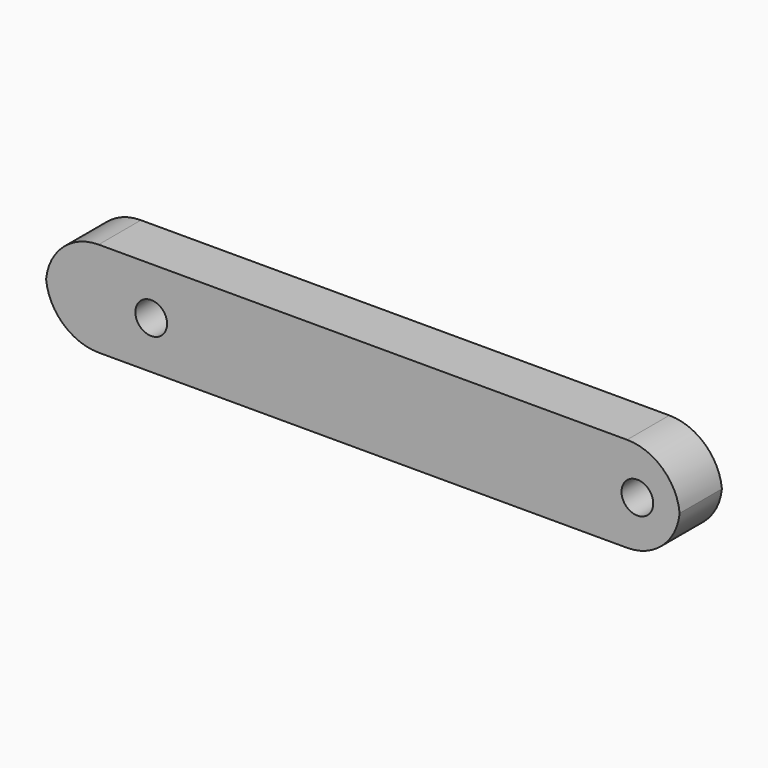
from build123d import *

# Parameters (mm, degrees)
F0_W        = 60
F0_H        = 9
F1_DEPTH    = 5
F2_T1_DEPTH = 30
F3_R        = 1.5
F4_DEPTH    = 12.5


# Not quite as in the source:
# - a fillet or chamfer that OpenCascade refuses, or shapes differently, is made with other operations: its cross-section is extruded or revolved along the edge and cut away or added


with BuildPart() as f1:
    # F0 (on Front) → F1 (new body)
    with BuildSketch(Plane.XZ):
        Rectangle(F0_W, F0_H)
    extrude(amount=F1_DEPTH)

    # F2: fillet of radius 5 on 4 edges, made by hand

    # F2_s2 → F2_t1 (cut)
    with BuildSketch(Plane.XZ.offset(-12.5)):
        with BuildLine():
            ThreePointArc((-25, 4.5), (-28.5355339059, 3.0355339059), (-30, -0.5))
            Line((-30, -0.5), (-30, 4.5))
            Line((-30, 4.5), (-25, 4.5))
        make_face()
        with BuildLine():
            ThreePointArc((-30, 0.5), (-28.5355339059, -3.0355339059), (-25, -4.5))
            Line((-25, -4.5), (-30, -4.5))
            Line((-30, -4.5), (-30, 0.5))
        make_face()
        with BuildLine():
            ThreePointArc((25, 4.5), (28.5355339059, 3.0355339059), (30, -0.5))
            Line((30, -0.5), (30, 4.5))
            Line((30, 4.5), (25, 4.5))
        make_face()
        with BuildLine():
            ThreePointArc((25, -4.5), (28.5355339059, -3.0355339059), (30, 0.5))
            Line((30, 0.5), (30, -4.5))
            Line((30, -4.5), (25, -4.5))
        make_face()
    extrude(amount=F2_T1_DEPTH, mode=Mode.SUBTRACT)

    # F3 (on Front) → F4 (cut, symmetric)
    with BuildSketch(Plane.XZ):
        with Locations((25.9749371855, 0)):
            Circle(F3_R)
        with Locations((-20.0250628145, 0)):
            Circle(F3_R)
    extrude(amount=F4_DEPTH, both=True, mode=Mode.SUBTRACT)


solid = f1.part
